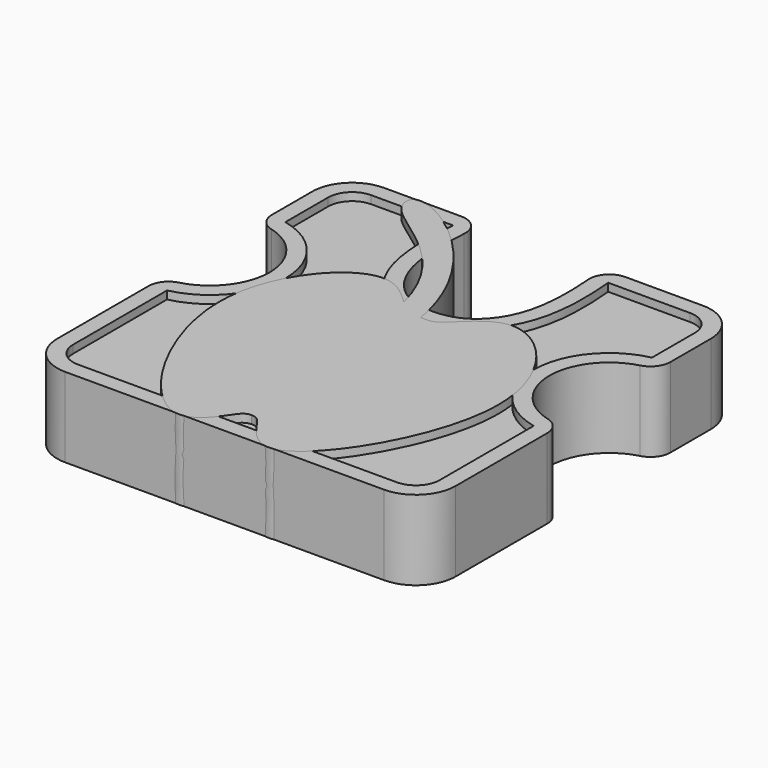
from build123d import *

# Parameters (mm, degrees)
F1_DEPTH = 2
F4_DEPTH = 0.2
F6_DEPTH = 2
F8_DEPTH = 2


# Not quite as in the source:
# - ends of sketch curves that miss each other by under 0.0002 mm in the source are joined
# - the dataset's text gives a spline's control points without its knots; the knots are read off the source's solid


with BuildPart() as f1:
    # F0 (on Top) → F1 (new body)
    with BuildSketch(Plane.XY):
        with BuildLine():
            Line((-2.0547145964, 5), (-4, 5))
            ThreePointArc((-4, 5), (-4.7071067812, 4.7071067812), (-5, 4))
            Line((-5, 4), (-5, 2.7339969853))
            ThreePointArc((-5, 2.7339969853), (-4.8960494593, 2.4288006128), (-4.6274206969, 2.2505055521))
            ThreePointArc((-4.6274206969, 2.2505055521), (-3.5096827878, 0.8000312525), (-4.6274206969, -0.6504430472))
            ThreePointArc((-4.6274206969, -0.6504430472), (-4.8960494593, -0.8287381079), (-5, -1.1339344804))
            Line((-5, -1.1339344804), (-5, -4))
            ThreePointArc((-5, -4), (-4.7071067812, -4.7071067812), (-4, -5))
            Line((-4, -5), (0, -5))
            Line((0, -5), (0, 1.5))
            add(Edge.make_bspline(
                [(-1.5563518663, 4.4595699461), (-1.665578556, 3.1131826426), (-1.3166269894, 1.9555787836), (-0.5056886543, 1.5), (0, 1.5)],
                knots=[0.068438024, 0.068438024, 0.068438024, 0.068438024, 0.6128012196, 1, 1, 1, 1], degree=3))
            ThreePointArc((-1.5563518663, 4.4595699461), (-1.6871448568, 4.8389579421), (-2.0547145964, 5))
        make_face()
    extrude(amount=F1_DEPTH)

    # F2: F1 across plane


with BuildPart() as f1_1:
    add(f1.part)
    add(f1.part.mirror(Plane.YZ))

    # F3 (on face) → F4 (cut)
    with BuildSketch(Plane.XY.offset(2)):
        with BuildLine():
            Line((-4.6, 4), (-4.6, 2.6553371608))
            ThreePointArc((-4.6, 2.6553371608), (-3.1096827878, 0.8000312525), (-4.6, -1.0552746559))
            Line((-4.6, -1.0552746559), (-4.6, -4))
            ThreePointArc((-4.6, -4), (-4.4242640687, -4.4242640687), (-4, -4.6))
            Line((-4, -4.6), (4, -4.6))
            ThreePointArc((4, -4.6), (4.4242640687, -4.4242640687), (4.6, -4))
            Line((4.6, -4), (4.6, -1.0552746559))
            ThreePointArc((4.6, -1.0552746559), (3.1096827878, 0.8000312525), (4.6, 2.6553371608))
            Line((4.6, 2.6553371608), (4.6, 4))
            ThreePointArc((4.6, 4), (4.4242640687, 4.4242640687), (4, 4.6))
            Line((4, 4.6), (1.9457486728, 4.6))
            add(Edge.make_bspline(
                [(1.9457486728, 4.6), (1.9925548829, 4.0867743279), (2.0010575411, 3.3808403194), (1.8726510373, 2.6225846563), (1.7053315953, 2.1896841722), (1.5289301657, 1.8971491367), (1.381220438, 1.706160192), (1.2130312765, 1.5329898835), (0.9536478928, 1.3299113304), (0.5628393096, 1.1474728371), (0.1954887297, 1.1), (0, 1.1)],
                knots=[0.0545601289, 0.0545601289, 0.0545601289, 0.0545601289, 0.25, 0.375, 0.5, 0.5625, 0.625, 0.6875, 0.75, 0.875, 1, 1, 1, 1], degree=3))
            add(Edge.make_bspline(
                [(0, 1.1), (-0.1954887297, 1.1), (-0.5628393096, 1.1474728371), (-0.9536478928, 1.3299113304), (-1.2130312765, 1.5329898835), (-1.381220438, 1.706160192), (-1.5289301657, 1.8971491367), (-1.7053315953, 2.1896841722), (-1.8726510373, 2.6225846563), (-2.0010575411, 3.3808403194), (-1.9925548829, 4.0867743279), (-1.9458318769, 4.6000075745)],
                knots=[0, 0, 0, 0, 0.125, 0.25, 0.3125, 0.375, 0.4375, 0.5, 0.625, 0.75, 0.9454398711, 0.9454398711, 0.9454398711, 0.9454398711], degree=3))
            Line((-1.9458318769, 4.6000075745), (-4, 4.6))
            ThreePointArc((-4, 4.6), (-4.4242640687, 4.4242640687), (-4.6, 4))
        make_face()
    extrude(amount=-F4_DEPTH, mode=Mode.SUBTRACT)


with BuildPart() as f6:
    # F5 (on Top) → F6 (new body)
    with BuildSketch(Plane.XY):
        with BuildLine():
            Line((0, -4.1498326625), (0, 1.1461564735))
            add(Edge.make_bspline(
                [(0, 1.1461564735), (-0.2331846159, 1.1461564735), (-0.3581305558, 1.1504604625), (-0.5919044569, 1.3833781015), (-0.6692804032, 1.4589919406)],
                knots=[0, 0, 0, 0, 0.0913485445, 0.1292998538, 0.1292998538, 0.1292998538, 0.1292998538], degree=3))
            add(Edge.make_bspline(
                [(-0.6692804032, 1.4589919406), (-0.9050007994, 1.6893442008), (-1.8762146695, 2.6011575331), (-4.7411558919, -0.6074326903), (-1.4634880482, -5.8912003005), (-0.34571211, -4.4574978545), (-0.171748246, -4.1498326625), (0, -4.1498326625)],
                knots=[0.1292998538, 0.1292998538, 0.1292998538, 0.1292998538, 0.2449158571, 0.4834978148, 0.775264767, 0.9095925993, 1, 1, 1, 1], degree=3))
        make_face()
    extrude(amount=F6_DEPTH)

    # F7: F6 across plane


with BuildPart() as f6_1:
    add(f6.part)
    add(f6.part.mirror(Plane.YZ))

    # F5 (on Top) → F8 (join)
    with BuildSketch(Plane.XY):
        with BuildLine():
            add(Edge.make_bspline(
                [(0, 1.1461564735), (-0.2331846159, 1.1461564735), (-0.3581305558, 1.1504604625), (-0.5919044569, 1.3833781015), (-0.6692804032, 1.4589919406)],
                knots=[0, 0, 0, 0, 0.0913485445, 0.1292998538, 0.1292998538, 0.1292998538, 0.1292998538], degree=3))
            add(Edge.make_bspline(
                [(-0.6692804032, 1.4589919406), (-1.1935472477, 3.5048075535), (-3.3214796159, 4.1185453251), (-3.3638279702, 5.6469634891), (-0.4057508777, 3.6138074938), (0, 1.1461564735)],
                knots=[0.0193878948, 0.0193878948, 0.0193878948, 0.0193878948, 0.4145137843, 0.551274714, 1, 1, 1, 1], degree=3))
        make_face()
    extrude(amount=F8_DEPTH)


solid = Compound([f1_1.part, f6_1.part])
